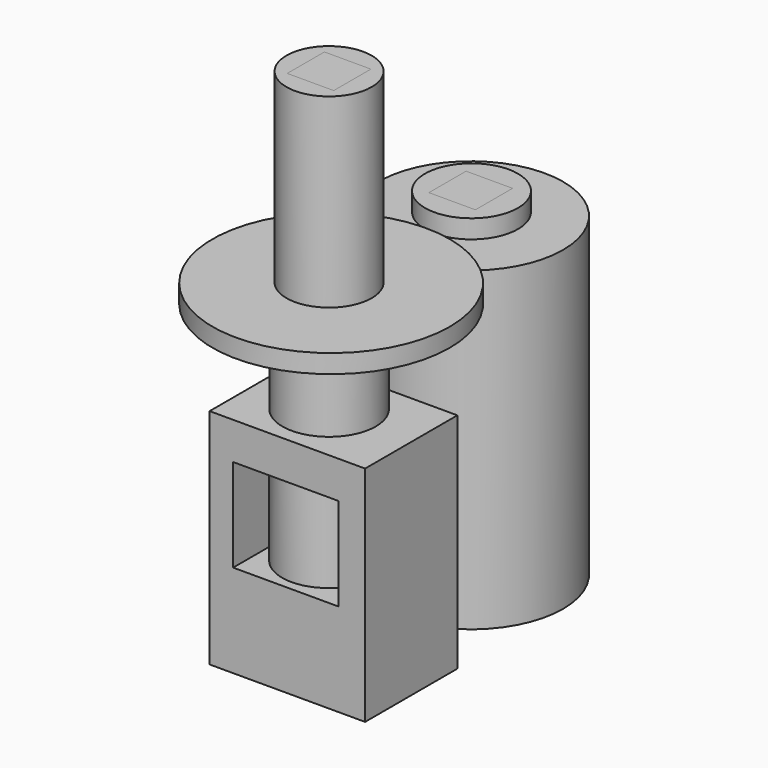
from build123d import *

# Parameters (mm, degrees)
F0_R      = 12.6238
F1_DEPTH  = 17.78
F0_R_2    = 4.2291
F2_R      = 6.376929238
F2_R_2    = 4.2291
F3_DEPTH  = 12.7
F4_W      = 21.2488458492
F4_H      = 15.7541136723
F5_DEPTH  = 5.08
F6_W      = 6.35
F6_H      = 6.35
F7_DEPTH  = 2.54
F8_W      = 6.35
F8_H      = 6.35
F9_DEPTH  = 3.048
F10_R     = 16.2146713523
F10_W     = 6.35
F10_H     = 6.35
F11_DEPTH = 2.54
F12_R     = 6.3530257629
F12_W     = 6.35
F12_H     = 6.35
F13_DEPTH = 2.54
F14_R     = 5.8220855013
F14_W     = 6.35
F14_H     = 6.35
F15_DEPTH = 25.4
F16_DEPTH = 25.4
F17_DEPTH = 19.05
F18_R     = 6.35
F19_DEPTH = 12.7
F20_W     = 3.6265931558
F20_H     = 15.7541136723
F20_W_2   = 3.216993995
F21_DEPTH = 25.4
F22_DEPTH = 6.35
F23_W     = 15.7541136723
F23_H     = 12.7
F24_DEPTH = 15.24


with BuildPart() as f1:
    # F0 (on Top) → F1 (new body)
    with BuildSketch(Plane.XY):
        with Locations((-6.3880984679, 32.7563181388)):
            Circle(F0_R)
    extrude(amount=F1_DEPTH)

    # F8 (on face) → F9 (join)
    with BuildSketch(Plane.XY.offset(17.78)):
        with Locations((-6.3880984679, 32.7563181388)):
            Rectangle(F8_W, F8_H)
    extrude(amount=F9_DEPTH)

    # F17 (add): a face of the model
    f17_faces = [f1.faces().sort_by_distance(p)[0] for p in [
        (-6.3880984679, 32.7563181388, 0),
    ]]
    extrude(f17_faces, amount=F17_DEPTH)

    # F22 (add): a face of the model
    f22_faces = [f1.faces().sort_by_distance(p)[0] for p in [
        (-6.3880984679, 32.7563181388, -19.05),
    ]]
    extrude(f22_faces, amount=F22_DEPTH)


with BuildPart() as f1b:
    # F0 (on Top) → F1, piece 2 (new body)
    with BuildSketch(Plane.XY):
        with Locations((-5.5065363796, 7.4605747914)):
            Circle(F0_R_2)
    extrude(amount=F1_DEPTH)

    # F2 (on face) → F3 (join)
    with BuildSketch(Plane.XY.offset(17.78)):
        with Locations((-5.5065363796, 7.4605747914)):
            Circle(F2_R)
        with Locations((-5.5065363796, 7.4605747914)):
            Circle(F2_R_2, mode=Mode.SUBTRACT)
    extrude(amount=-F3_DEPTH)

    # F4 (on Top) → F5 (join)
    with BuildSketch(Plane.XY):
        with Locations((-4.5697938185, 7.0365635911)):
            Rectangle(F4_W, F4_H)
    extrude(amount=F5_DEPTH)

    # F6 (on face) → F7 (join)
    with BuildSketch(Plane.XY.offset(17.78)):
        with Locations((-5.5334656176, 7.4875040295)):
            Rectangle(F6_W, F6_H)
    extrude(amount=F7_DEPTH)


with BuildPart() as f11:
    # F10 (on face) → F11 (new body)
    with BuildSketch(Plane.XY.offset(20.32)):
        with Locations((-5.289810244, 7.5345193036)):
            Circle(F10_R)
        with Locations((-5.5334656176, 7.4875040295)):
            Rectangle(F10_W, F10_H, mode=Mode.SUBTRACT)
    extrude(amount=-F11_DEPTH)

    # F14 (on face) → F15 (join)
    with BuildSketch(Plane.XY.offset(20.32)):
        with Locations((-5.5334656176, 7.4875040295)):
            Circle(F14_R)
        with Locations((-5.5334656176, 7.4875040295)):
            Rectangle(F14_W, F14_H, mode=Mode.SUBTRACT)
    extrude(amount=F15_DEPTH)


with BuildPart() as f13:
    # F12 (on face) → F13 (new body)
    with BuildSketch(Plane.XY.offset(20.828)):
        with Locations((-6.275807973, 32.7456742525)):
            Circle(F12_R)
        with Locations((-6.3880984679, 32.7563181388)):
            Rectangle(F12_W, F12_H, mode=Mode.SUBTRACT)
    extrude(amount=-F13_DEPTH)


with BuildPart() as f16:
    # F16 (new): a face of the model
    f16_faces = [f1b.part.faces().sort_by_distance(p)[0] for p in [
        (-5.5334656176, 7.4875040295, 20.32),
    ]]
    extrude(f16_faces, amount=F16_DEPTH)


with BuildPart() as f1b_1:
    add(f1b.part)

    # F18 (on face) → F19 (join)
    with BuildSketch(Plane(origin=(0, 0, 0), x_dir=(1, 0, 0), z_dir=(0, 0, -1))):
        with Locations((-5.0342167431, -6.7795067549)):
            Circle(F18_R)
    extrude(amount=F19_DEPTH)

    # F20 (on face) → F21 (join)
    with BuildSketch(Plane(origin=(0, 0, 0), x_dir=(1, 0, 0), z_dir=(0, 0, -1))):
        with Locations((4.2413325282, -7.0365635911)):
            Rectangle(F20_W, F20_H)
        with Locations((-13.5857197456, -7.0365635911)):
            Rectangle(F20_W_2, F20_H)
    extrude(amount=F21_DEPTH)

    # F23 (on face) → F24 (join)
    with BuildSketch(Plane(origin=(2.4280359503, 0, 0), x_dir=(0, -1, 0), z_dir=(-1, 0, 0))):
        with Locations((-7.0365635911, -19.05)):
            Rectangle(F23_W, F23_H)
    extrude(amount=F24_DEPTH)


solid = Compound([f1.part, f11.part, f13.part, f16.part, f1b_1.part])
